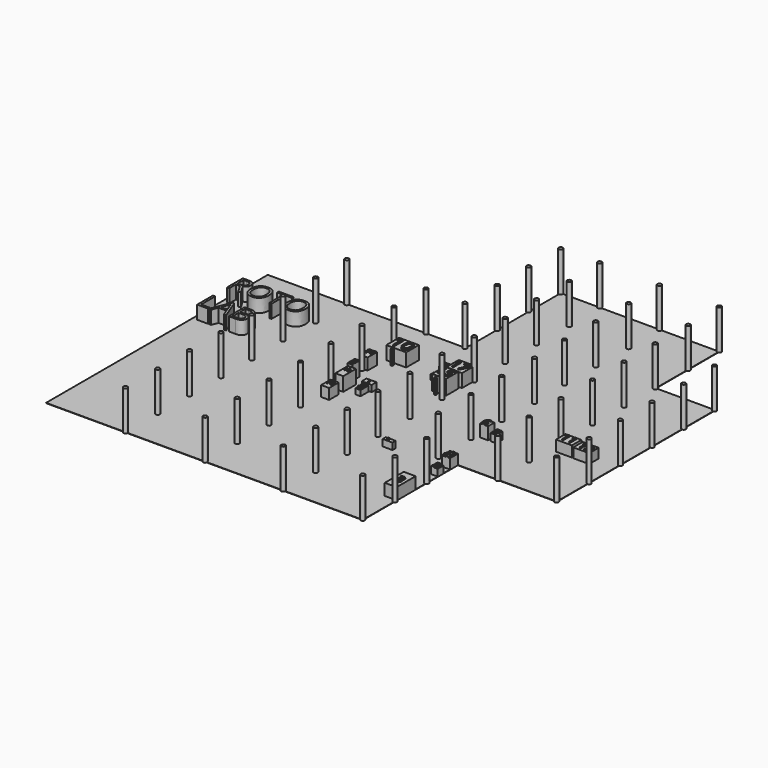
from build123d import *

# Parameters (mm, degrees)
F1_DEPTH      = 50.8
F2_TEXT_SIZE  = 4232.6821221246
F3_DEPTH      = 2057.4
F4_R          = 317.5
F5_DEPTH      = 6096
F6_W          = 1524
F6_H          = 914.4
F7_DEPTH      = 990.6
F9_W          = 1828.8
F9_H          = 3657.6
F10_DEPTH     = 1778
F11_W         = 1219.2
F11_H         = 1524
F12_DEPTH     = 1524
F13_W         = 1066.8
F13_H         = 1143
F14_DEPTH     = 1041.4
F15_W         = 1219.2
F15_H         = 1219.2
F16_DEPTH     = 1905
F17_W         = 914.4
F17_H         = 1219.2
F18_DEPTH     = 1092.2
F8_W          = 736.6
F8_H          = 1397
F19_DEPTH     = 2184.4
F20_W         = 787.4
F20_H         = 1524
F21_DEPTH     = 838.2
F22_W         = 1524
F22_H         = 609.6
F23_DEPTH     = 1016
F24_W         = 3048
F24_H         = 2438.4
F25_DEPTH     = 2057.4
F26_W         = 2438.4
F26_H         = 1828.8
F27_DEPTH     = 1651
F28_W         = 2438.4
F28_H         = 1828.8
F29_DEPTH     = 1473.2
F30_W         = 1219.2
F30_H         = 1828.8
F31_DEPTH     = 1778
F32_W         = 2133.6
F32_H         = 2438.4
F33_DEPTH     = 2286
F34_W         = 1524
F34_H         = 609.6
F35_DEPTH     = 762
F36_W         = 1219.2
F36_H         = 1828.8
F37_DEPTH     = 1625.6
F38_W         = 2438.4
F38_H         = 2438.4
F39_DEPTH     = 2032
F40_W         = 914.4
F40_H         = 1219.2
F41_DEPTH     = 1524
F42_W         = 254
F42_H         = 279.4
F43_DEPTH     = 2286
F44_W         = 279.4
F44_H         = 330.2
F45_DEPTH     = 2184.4
F46_TEXT_SIZE = 641.7221493191
F47_DEPTH     = 127
F48_TEXT_SIZE = 1140.0580406189
F49_DEPTH     = 127
F50_TEXT_SIZE = 1789.9645699395
F51_DEPTH     = 127
F52_TEXT_SIZE = 2005.52409416
F53_DEPTH     = 127
F54_TEXT_SIZE = 1587.5
F55_DEPTH     = 127
F56_TEXT_SIZE = 1693.3333333333
F57_DEPTH     = 127
F58_TEXT_SIZE = 1368.7968254089
F59_DEPTH     = 127
F60_TEXT_SIZE = 1526.7345640394
F61_DEPTH     = 127
F62_TEXT_SIZE = 623.5417392519
F63_DEPTH     = 127
F64_TEXT_SIZE = 2589.7873772515
F65_DEPTH     = 127
F66_TEXT_SIZE = 1862.5590536329
F67_DEPTH     = 127
F68_TEXT_SIZE = 1816.2886301676
F69_DEPTH     = 127
F70_TEXT_SIZE = 1151.0160234239
F71_DEPTH     = 127
F72_TEXT_SIZE = 2159.9425209893
F73_DEPTH     = 127
F74_TEXT_SIZE = 586.3149960836
F75_DEPTH     = 127
F76_TEXT_SIZE = 2159.129248725
F77_DEPTH     = 127
F78_TEXT_SIZE = 1074.8863220215
F79_DEPTH     = 127
F80_W         = 1219.2
F80_H         = 2438.4
F81_DEPTH     = 2133.6
F82_TEXT_SIZE = 798.2399728563
F83_DEPTH     = 127
F84_TEXT_SIZE = 375.6443659465
F85_DEPTH     = 127
F86_TEXT_SIZE = 186.7135365804
F87_DEPTH     = 127
F88_TEXT_SIZE = 194.2753791809
F89_DEPTH     = 127


# Not quite as in the source:
# - Text() gives the source's letters only with a copy of the font that has no kerning and outlines rounded to 1/6400 em; it was checked with that copy


with BuildPart() as f1:
    # F0 (on Top) → F1 (new body)
    with BuildSketch(Plane.XY):
        Polygon((15728.0017923199, -18288), (15728.0017923199, 0), (30968.0017923198, 0), (30968.0017923199, 30480), (21824.0017923199, 30480), (21824.0017923199, 42672), (-2559.9982076801, 42672), (-2559.9982076801, 24384), (-33039.9982076801, 24384), (-33039.9982076801, 0), (-33039.9982076801, -18288), align=None)
    extrude(amount=F1_DEPTH)

    # F4 (on face) → F5 (join)
    with BuildSketch(Plane.XY.offset(50.8)):
        with Locations((-20799.596786499, 6015.6626701355)):
            Circle(F4_R)
        with Locations((-20946.6915130615, 12207.6358795166)):
            Circle(F4_R)
        with Locations((-20800.8155822754, 18305.2234649658)):
            Circle(F4_R)
        with Locations((-20859.1651916504, 24373.6362457275)):
            Circle(F4_R)
        with Locations((-8556.0779571533, 84.7052112222)):
            Circle(F4_R)
        with Locations((-8721.1170196533, 6149.890422821)):
            Circle(F4_R)
        with Locations((-8762.3767852783, 12173.8157272339)):
            Circle(F4_R)
        with Locations((-8721.1170196533, 18280.2619934082)):
            Circle(F4_R)
        with Locations((-8638.5974884033, 24345.4475402832)):
            Circle(F4_R)
        with Locations((-2655.9314727783, 24345.4475402832)):
            Circle(F4_R)
        with Locations((-2532.1514606476, 30410.6330871582)):
            Circle(F4_R)
        with Locations((-2614.6714687347, 36558.3381652832)):
            Circle(F4_R)
        with Locations((-2532.1526527405, 42623.5237121582)):
            Circle(F4_R)
        with Locations((3409.2543125153, 42706.0432434082)):
            Circle(F4_R)
        with Locations((3574.2921829224, 36640.8576965332)):
            Circle(F4_R)
        with Locations((3491.7731285095, 30451.8928527832)):
            Circle(F4_R)
        with Locations((3574.2919445038, 24304.1896820068)):
            Circle(F4_R)
        with Locations((3656.8119525909, 18239.0041351318)):
            Circle(F4_R)
        with Locations((3491.7728900909, 12256.3371658325)):
            Circle(F4_R)
        with Locations((3574.2919445038, 5984.8532676697)):
            Circle(F4_R)
        with Locations((3491.7728900909, -80.3316086531)):
            Circle(F4_R)
        with Locations((12733.9611053467, 2.1870692726)):
            Circle(F4_R)
        with Locations((12733.9611053467, 6273.6721038818)):
            Circle(F4_R)
        with Locations((12692.7003860474, 12256.3371658325)):
            Circle(F4_R)
        with Locations((12816.4787292481, 18404.0431976318)):
            Circle(F4_R)
        with Locations((12651.4387130737, 24386.7073059082)):
            Circle(F4_R)
        with Locations((12651.4387130737, 30410.6330871582)):
            Circle(F4_R)
        with Locations((12752.1867752075, 36600.887298584)):
            Circle(F4_R)
        with Locations((12653.694152832, 42639.289855957)):
            Circle(F4_R)
        with Locations((21813.2495880127, 42717.7085876465)):
            Circle(F4_R)
        with Locations((21886.848449707, 36633.472442627)):
            Circle(F4_R)
        with Locations((21813.2514953613, 30402.042388916)):
            Circle(F4_R)
        with Locations((30964.1361236572, 30352.9758453369)):
            Circle(F4_R)
        with Locations((21837.7838134766, 24366.8746948242)):
            Circle(F4_R)
        with Locations((21788.7172698975, 18331.7070007324)):
            Circle(F4_R)
        with Locations((31013.2007598877, 24366.8746948242)):
            Circle(F4_R)
        with Locations((30988.6684417725, 18307.1727752686)):
            Circle(F4_R)
        with Locations((21886.8503570557, 12173.8739013672)):
            Circle(F4_R)
        with Locations((30964.1342163086, 12247.4727630615)):
            Circle(F4_R)
        with Locations((21862.3161315918, 6065.1059150696)):
            Circle(F4_R)
        with Locations((31013.2007598877, 6163.2390022278)):
            Circle(F4_R)
        with Locations((21911.3826751709, -19.1279165447)):
            Circle(F4_R)
        with Locations((30939.6018981934, 5.4047219455)):
            Circle(F4_R)
        with Locations((-20793.7927246094, 82.6025158167)):
            Circle(F4_R)
        with Locations((-20807.9624176025, -5984.0641021729)):
            Circle(F4_R)
        with Locations((-20780.4508209229, -12108.3498001099)):
            Circle(F4_R)
        with Locations((-20805.7613372803, -18297.191619873)):
            Circle(F4_R)
        with Locations((-8567.421913147, -5956.3798904419)):
            Circle(F4_R)
        with Locations((-8567.421913147, -12081.9406509399)):
            Circle(F4_R)
        with Locations((-8553.3752441406, -18285.0437164307)):
            Circle(F4_R)
        with Locations((3495.8996772766, -18306.324005127)):
            Circle(F4_R)
        with Locations((3490.2019500732, -12072.8397369385)):
            Circle(F4_R)
        with Locations((3511.4879608154, -6029.2134284973)):
            Circle(F4_R)
        with Locations((15735.5194091797, -5993.4167861938)):
            Circle(F4_R)
        with Locations((15717.6218032837, -12096.7893600464)):
            Circle(F4_R)
        with Locations((15699.7241973877, -18253.8547515869)):
            Circle(F4_R)
    extrude(amount=F5_DEPTH)


with BuildPart() as f3:
    # F2 (on face) → F3 (new body)
    with BuildSketch(Plane.XY.offset(50.8)):
        with Locations((-32772.6535797119, 15699.7089385986)):
            Text('ROTO', F2_TEXT_SIZE, font='Open Sans', text_align=(TextAlign.LEFT, TextAlign.BOTTOM))
        with Locations((-32772.6535797119, 9943.2612525092)):
            Text('LAB', F2_TEXT_SIZE, font='Open Sans', text_align=(TextAlign.LEFT, TextAlign.BOTTOM))
    extrude(amount=F3_DEPTH)


with BuildPart() as f7:
    # F6 (on face) → F7 (new body)
    with BuildSketch(Plane.XY.offset(50.8)):
        with Locations((-4957.612991333, 8778.4770334664)):
            Rectangle(F6_W, F6_H)
    extrude(amount=F7_DEPTH)

    # F46 (on face) → F47 (join)
    with BuildSketch(Plane.XY.offset(1041.4)):
        with Locations((-5127.6893615723, 8515.8033370972)):
            Text('1', F46_TEXT_SIZE, font='Open Sans', font_style=FontStyle.BOLD, text_align=(TextAlign.LEFT, TextAlign.BOTTOM))
    extrude(amount=F47_DEPTH)


with BuildPart() as f10:
    # F9 (on face) → F10 (new body)
    with BuildSketch(Plane.XY.offset(50.8)):
        with Locations((14813.6017923199, -9950.6590812711)):
            Rectangle(F9_W, F9_H)
    extrude(amount=F10_DEPTH)

    # F50 (on face) → F51 (join)
    with BuildSketch(Plane.XY.offset(1828.8)):
        with Locations((14328.556060791, -10550.2853393555)):
            Text('3', F50_TEXT_SIZE, font='Open Sans', font_style=FontStyle.BOLD, text_align=(TextAlign.LEFT, TextAlign.BOTTOM))
    extrude(amount=F51_DEPTH)


with BuildPart() as f12:
    # F11 (on face) → F12 (new body)
    with BuildSketch(Plane.XY.offset(50.8)):
        with Locations((15118.4017923199, -762)):
            Rectangle(F11_W, F11_H)
    extrude(amount=F12_DEPTH)

    # F52 (on face) → F53 (join)
    with BuildSketch(Plane.XY.offset(1574.8)):
        with Locations((14484.5768539407, -1524)):
            Text('4', F52_TEXT_SIZE, font='Open Sans', font_style=FontStyle.BOLD, text_align=(TextAlign.LEFT, TextAlign.BOTTOM))
    extrude(amount=F53_DEPTH)


with BuildPart() as f14:
    # F13 (on face) → F14 (new body)
    with BuildSketch(Plane.XY.offset(50.8)):
        with Locations((15194.6017923199, -3302.9518756866)):
            Rectangle(F13_W, F13_H)
    extrude(amount=F14_DEPTH)

    # F54 (on face) → F55 (join)
    with BuildSketch(Plane.XY.offset(1092.2)):
        with Locations((14661.2017923199, -3874.4518756866)):
            Text('5', F54_TEXT_SIZE, font='Open Sans', font_style=FontStyle.BOLD, text_align=(TextAlign.LEFT, TextAlign.BOTTOM))
    extrude(amount=F55_DEPTH)


with BuildPart() as f16:
    # F15 (on face) → F16 (new body)
    with BuildSketch(Plane.XY.offset(50.8)):
        with Locations((13953.0682563782, 7881.6367265476)):
            Rectangle(F15_W, F15_H)
    extrude(amount=F16_DEPTH)


with BuildPart() as f18:
    # F17 (on face) → F18 (new body)
    with BuildSketch(Plane.XY.offset(50.8)):
        with Locations((15360.1171970367, 7915.4676161204)):
            Rectangle(F17_W, F17_H)
    extrude(amount=F18_DEPTH)


with BuildPart() as f19:
    # F8 (on face) → F19 (new body)
    with BuildSketch(Plane.XY.offset(50.8)):
        with Locations((-8222.0997810364, 9870.9979331705)):
            Rectangle(F8_W, F8_H)
    extrude(amount=F19_DEPTH)


with BuildPart() as f21:
    # F20 (on face) → F21 (new body)
    with BuildSketch(Plane.XY.offset(50.8)):
        with Locations((-4968.0386975248, 7420.0875759125)):
            Rectangle(F20_W, F20_H)
    extrude(amount=F21_DEPTH)


with BuildPart() as f23:
    # F22 (on face) → F23 (new body)
    with BuildSketch(Plane.XY.offset(50.8)):
        with Locations((6423.1383800507, -1579.3040680206)):
            Rectangle(F22_W, F22_H)
    extrude(amount=F23_DEPTH)


with BuildPart() as f25:
    # F24 (on face) → F25 (new body)
    with BuildSketch(Plane.XY.offset(50.8)):
        with Locations((-6495.6240653992, 17147.1932375824)):
            Rectangle(F24_W, F24_H)
    extrude(amount=F25_DEPTH)


with BuildPart() as f27:
    # F26 (on face) → F27 (new body)
    with BuildSketch(Plane.XY.offset(50.8)):
        with Locations((24011.1246109009, 10985.4101134314)):
            Rectangle(F26_W, F26_H)
    extrude(amount=F27_DEPTH)


with BuildPart() as f29:
    # F28 (on face) → F29 (new body)
    with BuildSketch(Plane.XY.offset(50.8)):
        with Locations((26698.148727417, 10952.7915389094)):
            Rectangle(F28_W, F28_H)
    extrude(amount=F29_DEPTH)


with BuildPart() as f31:
    # F30 (on face) → F31 (new body)
    with BuildSketch(Plane.XY.offset(50.8)):
        with Locations((-8701.7737822697, 13314.9287807601)):
            Rectangle(F30_W, F30_H)
    extrude(amount=F31_DEPTH)


with BuildPart() as f33:
    # F32 (on face) → F33 (new body)
    with BuildSketch(Plane.XY.offset(50.8)):
        with Locations((2291.647195816, 14386.6032997991)):
            Rectangle(F32_W, F32_H)
    extrude(amount=F33_DEPTH)

    # F72 (on face) → F73 (join)
    with BuildSketch(Plane.XY.offset(2336.8)):
        with Locations((986.518740654, 13797.9917526245)):
            Text('15', F72_TEXT_SIZE, font='Open Sans', text_align=(TextAlign.LEFT, TextAlign.BOTTOM))
    extrude(amount=F73_DEPTH)


with BuildPart() as f35:
    # F34 (on face) → F35 (new body)
    with BuildSketch(Plane.XY.offset(50.8)):
        with Locations((90.006724, 15543.237889696)):
            Rectangle(F34_W, F34_H)
    extrude(amount=F35_DEPTH)


with BuildPart() as f37:
    # F36 (on face) → F37 (new body)
    with BuildSketch(Plane.XY.offset(50.8)):
        with Locations((-7536.473274231, 4466.957287801)):
            Rectangle(F36_W, F36_H)
    extrude(amount=F37_DEPTH)

    # F78 (on face) → F79 (join)
    with BuildSketch(Plane.XY.offset(1676.4)):
        with Locations((-8188.4775161743, 4304.6984672546)):
            Text('18', F78_TEXT_SIZE, font='Open Sans', text_align=(TextAlign.LEFT, TextAlign.BOTTOM))
    extrude(amount=F79_DEPTH)


with BuildPart() as f39:
    # F38 (on face) → F39 (new body)
    with BuildSketch(Plane.XY.offset(50.8)):
        with Locations((2396.9045877457, 17155.8533382776)):
            Rectangle(F38_W, F38_H)
    extrude(amount=F39_DEPTH)

    # F76 (on face) → F77 (join)
    with BuildSketch(Plane.XY.offset(2082.8)):
        with Locations((1103.9004325867, 16424.747467041)):
            Text('17', F76_TEXT_SIZE, font='Open Sans', text_align=(TextAlign.LEFT, TextAlign.BOTTOM))
    extrude(amount=F77_DEPTH)


with BuildPart() as f41:
    # F40 (on face) → F41 (new body)
    with BuildSketch(Plane.XY.offset(50.8)):
        with Locations((169.9298024178, 16984.8510244027)):
            Rectangle(F40_W, F40_H)
    extrude(amount=F41_DEPTH)


with BuildPart() as f43:
    # F42 (on face) → F43 (new body)
    with BuildSketch(Plane.XY.offset(50.8)):
        with Locations((2175.8086949678, 12656.8779945374)):
            Rectangle(F42_W, F42_H)
    extrude(amount=F43_DEPTH)


with BuildPart() as f45:
    # F44 (on face) → F45 (new body)
    with BuildSketch(Plane.XY.offset(50.8)):
        with Locations((-6676.3458251953, 15343.0423209322)):
            Rectangle(F44_W, F44_H)
    extrude(amount=F45_DEPTH)


with BuildPart() as f49:
    # F48 (on face) → F49 (new body)
    with BuildSketch(Plane.XY.offset(2235.2)):
        with Locations((-8467.2031402588, 9436.5978240967)):
            Text('2', F48_TEXT_SIZE, font='Open Sans', font_style=FontStyle.BOLD, text_align=(TextAlign.LEFT, TextAlign.BOTTOM))
    extrude(amount=F49_DEPTH)


with BuildPart() as f57:
    # F56 (on face) → F57 (new body)
    with BuildSketch(Plane.XY.offset(1955.8)):
        with Locations((13343.4682563782, 7272.0367265476)):
            Text('6', F56_TEXT_SIZE, font='Open Sans', text_align=(TextAlign.LEFT, TextAlign.BOTTOM))
    extrude(amount=F57_DEPTH)


with BuildPart() as f59:
    # F58 (on face) → F59 (new body)
    with BuildSketch(Plane.XY.offset(1143)):
        with Locations((14999.5145797729, 7429.0294647217)):
            Text('7', F58_TEXT_SIZE, font='Open Sans', text_align=(TextAlign.LEFT, TextAlign.BOTTOM))
    extrude(amount=F59_DEPTH)


with BuildPart() as f61:
    # F60 (on face) → F61 (new body)
    with BuildSketch(Plane.XY.offset(889)):
        with Locations((-5426.9428253174, 6873.2976913452)):
            Text('8', F60_TEXT_SIZE, font='Open Sans', text_align=(TextAlign.LEFT, TextAlign.BOTTOM))
    extrude(amount=F61_DEPTH)


with BuildPart() as f63:
    # F62 (on face) → F63 (new body)
    with BuildSketch(Plane.XY.offset(1066.8)):
        with Locations((6085.7753753662, -1783.7051153183)):
            Text('9', F62_TEXT_SIZE, font='Open Sans', text_align=(TextAlign.LEFT, TextAlign.BOTTOM))
    extrude(amount=F63_DEPTH)


with BuildPart() as f65:
    # F64 (on face) → F65 (new body)
    with BuildSketch(Plane.XY.offset(2108.2)):
        with Locations((-7991.6224479675, 16297.4281311035)):
            Text('10', F64_TEXT_SIZE, font='Open Sans', text_align=(TextAlign.LEFT, TextAlign.BOTTOM))
    extrude(amount=F65_DEPTH)


with BuildPart() as f67:
    # F66 (on face) → F67 (new body)
    with BuildSketch(Plane.XY.offset(1701.8)):
        with Locations((22940.7768249512, 10429.0227890015)):
            Text('11', F66_TEXT_SIZE, font='Open Sans', text_align=(TextAlign.LEFT, TextAlign.BOTTOM))
    extrude(amount=F67_DEPTH)


with BuildPart() as f69:
    # F68 (on face) → F69 (new body)
    with BuildSketch(Plane.XY.offset(1524)):
        with Locations((25713.6974334717, 10347.2805023193)):
            Text('12', F68_TEXT_SIZE, font='Open Sans', text_align=(TextAlign.LEFT, TextAlign.BOTTOM))
    extrude(amount=F69_DEPTH)


with BuildPart() as f71:
    # F70 (on face) → F71 (new body)
    with BuildSketch(Plane.XY.offset(1828.8)):
        with Locations((-9379.0049552917, 13243.7162399292)):
            Text('14', F70_TEXT_SIZE, font='Open Sans', text_align=(TextAlign.LEFT, TextAlign.BOTTOM))
    extrude(amount=F71_DEPTH)


with BuildPart() as f75:
    # F74 (on face) → F75 (new body)
    with BuildSketch(Plane.XY.offset(812.8)):
        with Locations((-160.5785489082, 15360.4431152344)):
            Text('16', F74_TEXT_SIZE, font='Open Sans', text_align=(TextAlign.LEFT, TextAlign.BOTTOM))
    extrude(amount=F75_DEPTH)


with BuildPart() as f81:
    # F80 (on face) → F81 (new body)
    with BuildSketch(Plane.XY.offset(50.8)):
        with Locations((-7525.1216492193, 7471.889257431)):
            Rectangle(F80_W, F80_H)
    extrude(amount=F81_DEPTH)

    # F82 (on face) → F83 (join)
    with BuildSketch(Plane.XY.offset(2184.4)):
        with Locations((-8002.6526451111, 7528.2378196716)):
            Text('19', F82_TEXT_SIZE, font='Open Sans', text_align=(TextAlign.LEFT, TextAlign.BOTTOM))
    extrude(amount=F83_DEPTH)


with BuildPart() as f85:
    # F84 (on face) → F85 (new body)
    with BuildSketch(Plane.XY.offset(1574.8)):
        with Locations((19.8181122541, 16975.4199981689)):
            Text('20', F84_TEXT_SIZE, font='Open Sans', text_align=(TextAlign.LEFT, TextAlign.BOTTOM))
    extrude(amount=F85_DEPTH)


with BuildPart() as f87:
    # F86 (on face) → F87 (new body)
    with BuildSketch(Plane.XY.offset(2336.8)):
        with Locations((2101.1898517609, 12612.6403808594)):
            Text('21', F86_TEXT_SIZE, font='Open Sans', text_align=(TextAlign.LEFT, TextAlign.BOTTOM))
    extrude(amount=F87_DEPTH)


with BuildPart() as f89:
    # F88 (on face) → F89 (new body)
    with BuildSketch(Plane.XY.offset(2235.2)):
        with Locations((-6789.1407012939, 15296.8454360962)):
            Text('22', F88_TEXT_SIZE, font='Open Sans', text_align=(TextAlign.LEFT, TextAlign.BOTTOM))
    extrude(amount=F89_DEPTH)


solid = Compound([f1.part, f3.part, f7.part, f10.part, f12.part, f14.part, f16.part, f18.part, f19.part, f21.part, f23.part, f25.part, f27.part, f29.part, f31.part, f33.part, f35.part, f37.part, f39.part, f41.part, f43.part, f45.part, f49.part, f57.part, f59.part, f61.part, f63.part, f65.part, f67.part, f69.part, f71.part, f75.part, f81.part, f85.part, f87.part, f89.part])
